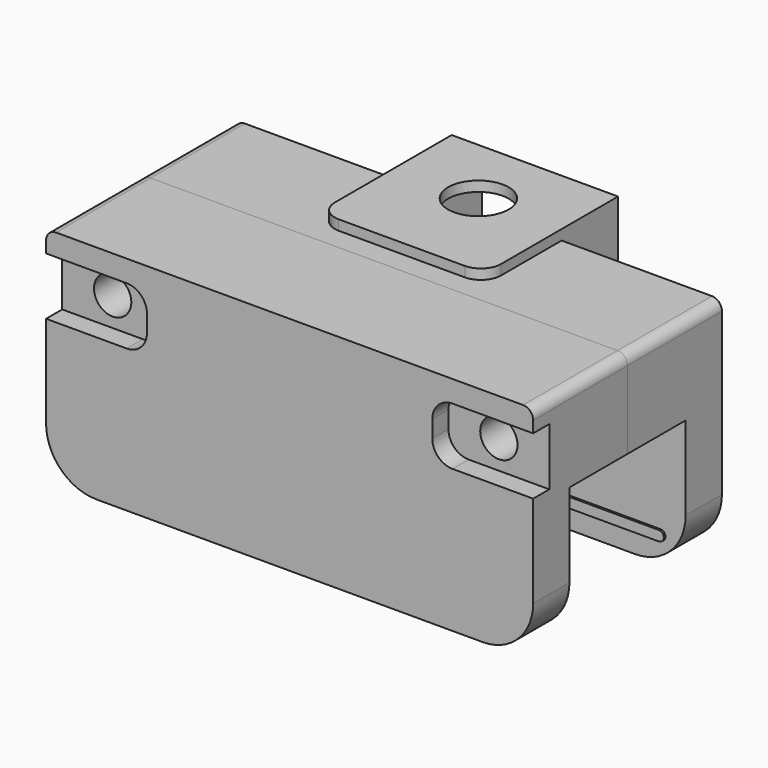
from build123d import *

# Parameters (mm, degrees)
F2_DEPTH        = 7.2
F3_W            = 48.3
F3_H            = 22
F4_DEPTH        = 4.5
F7_DEPTH        = 0.2
F10_D           = 3.7
F10_CBORE_D     = 6.5
F10_CBORE_DEPTH = 3
F11_D           = 3.7
F13_DEPTH       = 2
F14_R           = 1
F14_2_R         = 1
F15_R           = 5
F15_2_R         = 5
F17_DEPTH       = 5.5
F18_R           = 3
F19_DEPTH       = 1
F21_DEPTH       = 3


# Not quite as in the source:
# - a pattern or mirror of a feature is missing from the dataset's text; its kind, count and spacing are read off the source's solid


with BuildPart() as f2:
    # F1 (on Front) → F2 (new body)
    with BuildSketch(Plane.XZ):
        Polygon((-24.15, 0), (-24.15, -8.7), (-2.85, -8.7), (0, -11.55), (2.85, -8.7), (24.15, -8.7), (24.15, 0), align=None)
    extrude(amount=-F2_DEPTH)

    # F3 (on face) → F4 (join)
    with BuildSketch(Plane(origin=(0, 7.2, 0), x_dir=(-1, 0, 0), z_dir=(0, 1, 0))):
        with Locations((0, -11)):
            Rectangle(F3_W, F3_H)
    extrude(amount=F4_DEPTH)

    # F6 (on face) → F7 (join)
    with BuildSketch(Plane.XZ.offset(-7.2)):
        with BuildLine():
            ThreePointArc((22.15, -19.5), (22.0035533906, -19.1464466094), (21.65, -19))
            Line((21.65, -19), (-21.65, -19))
            ThreePointArc((-21.65, -19), (-22.0035533906, -19.1464466094), (-22.15, -19.5))
            ThreePointArc((-22.15, -19.5), (-22.0035533906, -19.8535533906), (-21.65, -20))
            Line((-21.65, -20), (21.65, -20))
            ThreePointArc((21.65, -20), (22.0035533906, -19.8535533906), (22.15, -19.5))
        make_face()
    extrude(amount=F7_DEPTH)


with BuildPart() as f8_1:
    # F8: instance of F2
    add(f2.part.mirror(Plane.XZ))

    # F11 (through all)
    with Locations(Plane.XZ.offset(11.7)):
        with Locations((-19.15, -5), (19.15, -5)):
            Hole(F11_D / 2)

    # F12 (on face) → F13 (cut)
    with BuildSketch(Plane.XZ.offset(11.7)):
        with BuildLine():
            Line((-16.15, -2.15), (-24.15, -2.15))
            Line((-24.15, -2.15), (-24.15, -7.85))
            Line((-24.15, -7.85), (-16.15, -7.85))
            ThreePointArc((-16.15, -7.85), (-14.7357864376, -7.2642135624), (-14.15, -5.85))
            Line((-14.15, -5.85), (-14.15, -4.15))
            ThreePointArc((-14.15, -4.15), (-14.7357864376, -2.7357864376), (-16.15, -2.15))
        make_face()
        with BuildLine():
            ThreePointArc((16.15, -2.15), (14.7357864376, -2.7357864376), (14.15, -4.15))
            Line((14.15, -4.15), (14.15, -5.85))
            ThreePointArc((14.15, -5.85), (14.7357864376, -7.2642135624), (16.15, -7.85))
            Line((16.15, -7.85), (24.15, -7.85))
            Line((24.15, -7.85), (24.15, -2.15))
            Line((24.15, -2.15), (16.15, -2.15))
        make_face()
    extrude(amount=-F13_DEPTH, mode=Mode.SUBTRACT)

    # F14#2
    f14_2_edges = [f8_1.edges().sort_by_distance(p)[0] for p in [
        (-24.15, -5.85, 0),
        (24.15, -5.85, 0),
    ]]
    fillet(f14_2_edges, radius=F14_2_R)

    # F15#2
    f15_2_edges = [f8_1.edges().sort_by_distance(p)[0] for p in [
        (24.15, -9.45, -22),
        (-24.15, -9.45, -22),
    ]]
    fillet(f15_2_edges, radius=F15_2_R)


with BuildPart() as f2_1:
    add(f2.part)

    # F10 (through all)
    with Locations(Plane(origin=(0, 11.7, 0), x_dir=(-1, 0, 0), z_dir=(0, 1, 0))):
        with Locations((-19.15, -5), (19.15, -5)):
            CounterBoreHole(F10_D / 2, F10_CBORE_D / 2, F10_CBORE_DEPTH)

    # F14
    f14_edges = [f2_1.edges().sort_by_distance(p)[0] for p in [
        (-24.15, 5.85, 0),
        (24.15, 5.85, 0),
    ]]
    fillet(f14_edges, radius=F14_R)

    # F15
    f15_edges = [f2_1.edges().sort_by_distance(p)[0] for p in [
        (24.15, 9.45, -22),
        (-24.15, 9.45, -22),
    ]]
    fillet(f15_edges, radius=F15_R)

    # F16 (on face) → F17 (cut)
    with BuildSketch(Plane.XY):
        with BuildLine():
            ThreePointArc((-5.25, 7.2), (-4.6642135624, 5.7857864376), (-3.25, 5.2))
            Line((-3.25, 5.2), (3.25, 5.2))
            ThreePointArc((3.25, 5.2), (4.6642135624, 5.7857864376), (5.25, 7.2))
            Line((5.25, 7.2), (5.25, 11.7))
            Line((5.25, 11.7), (-5.25, 11.7))
            Line((-5.25, 11.7), (-5.25, 7.2))
        make_face()
    extrude(amount=-F17_DEPTH, mode=Mode.SUBTRACT)

    # F18 (on face) → F19 (join)
    with BuildSketch(Plane.XY):
        with BuildLine():
            Line((8.25, 18.7), (-8.25, 18.7))
            Line((-8.25, 18.7), (-8.25, 4.2))
            ThreePointArc((-8.25, 4.2), (-7.6642135624, 2.7857864376), (-6.25, 2.2))
            Line((-6.25, 2.2), (6.25, 2.2))
            ThreePointArc((6.25, 2.2), (7.6642135624, 2.7857864376), (8.25, 4.2))
            Line((8.25, 4.2), (8.25, 18.7))
        make_face()
        with Locations((0, 11.7)):
            Circle(F18_R, mode=Mode.SUBTRACT)
    extrude(amount=F19_DEPTH)

    # F20 (on face) → F21 (join)
    with BuildSketch(Plane.YZ.offset(8.25)):
        with BuildLine():
            Line((18.7, -6.5), (18.7, 0))
            Line((18.7, 0), (11.7, 0))
            Line((11.7, 0), (11.7, -7.5))
            Line((11.7, -7.5), (17.7, -7.5))
            ThreePointArc((17.7, -7.5), (18.4071067812, -7.2071067812), (18.7, -6.5))
        make_face()
    f21 = extrude(amount=-F21_DEPTH)

    # F21_copies: F21 across plane
    add(f21.mirror(Plane(origin=(0, 0, 0), x_dir=(0, 0, -1), z_dir=(-1, 0, 0))))


solid = Compound([f8_1.part, f2_1.part])
